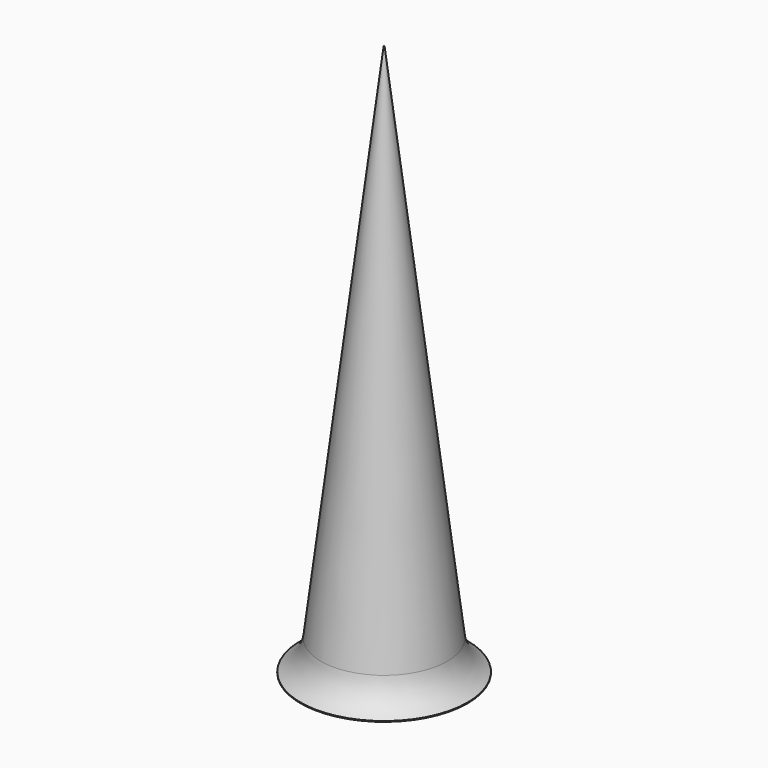
from build123d import *

# Parameters (mm, degrees)
F0_R     = 85
F2_R     = 0.5
F4_R     = 105.9677495378
F5_DEPTH = 1


# Not quite as in the source:
# - a fillet or chamfer that OpenCascade refuses, or shapes differently, is made with other operations: its cross-section is extruded or revolved along the edge and cut away or added


with BuildPart() as f3:
    # F0 (on Top) → F3 section 0
    with BuildSketch(Plane.XY):
        Circle(F0_R)
    # F2 (on offset) → F3 section 1
    with BuildSketch(Plane.XY.offset(700)):
        Circle(F2_R)
    loft()

    # F4 (on Top) → F5 (join)
    with BuildSketch(Plane.XY):
        Circle(F4_R)
    extrude(amount=F5_DEPTH)

    # F6: fillet of radius 50 on 1 edges, made by hand


with BuildPart() as f6_tool2:
    # F6_s3 → F6_t4 (revolve)
    with BuildSketch(Plane.XZ):
        with BuildLine():
            ThreePointArc((105.9675577084, 0.9996489993), (88.5489126941, 16.8340527655), (80.3057755127, 38.8837290936))
            Line((80.3057755127, 38.8837290936), (75.3416542323, 38.284488739))
            ThreePointArc((75.3416542323, 38.284488739), (77.6286078916, 19.3426481611), (79.9151644339, 0.4007596454))
            Line((79.9151644339, 0.4007596454), (84.8792857143, -4.0001589064))
            ThreePointArc((84.8792857143, -4.0001589064), (95.4234217114, -4.0001589064), (103.5696146476, -3.3879993647))
            Line((103.5696146476, -3.3879993647), (105.9675577084, 0.9996489993))
        make_face()
    revolve(axis=Axis((0, 0, 1), (0, 0, 1)))

    split(bisect_by=Plane.XY, keep=Keep.TOP)


with BuildPart() as f3_1:
    add(f3.part)

    # F6_t1: union F6_tool2
    add(f6_tool2.part)


solid = f3_1.part
